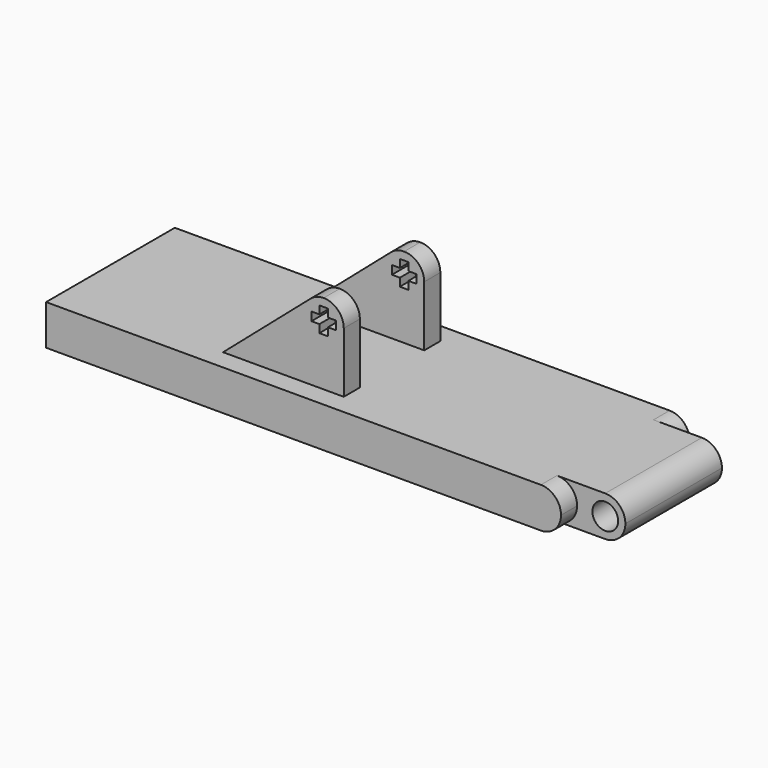
from build123d import *

# Parameters (mm, degrees)
F0_W     = 9.525
F0_H     = 23.8125
F1_DEPTH = 7.9375
F2_R     = 3.96874
F3_W     = 23.8125
F3_H     = 3.96875
F4_DEPTH = 15.875
F5_W     = 1.6891
F5_H     = 1.56845
F5_H_2   = 1.6891
F5_W_2   = 1.56845
F5_R     = 2.54
F6_DEPTH = 31.75


# Not quite as in the source:
# - a fillet or chamfer is up to 0.001 mm smaller than in the source, because OpenCascade refuses the exact size


with BuildPart() as f1:
    # F0 (on Top) → F1 (new body)
    with BuildSketch(Plane.XY):
        with Locations((-4.7625, -11.90625)):
            Rectangle(F0_W, F0_H)
        Polygon((-9.525, -23.8125), (-9.525, 0), (-9.525, 3.96875), (-111.125, 3.96875), (-111.125, -27.78125), (-9.525, -27.78125), align=None)
    extrude(amount=F1_DEPTH)

    # F2 (radius 3.96875 in the source; OpenCascade refuses exactly that, so slightly less here)
    f2_edges = [f1.edges().sort_by_distance(p)[0] for p in [
        (-9.525, -25.796875, 7.9375),
        (-9.525, -25.796875, 0),
        (0, -11.90625, 7.9375),
        (0, -11.90625, 0),
        (-9.525, 1.984375, 7.9375),
        (-9.525, 1.984375, 0),
    ]]
    fillet(f2_edges, radius=F2_R)

    # F3 (on face) → F4 (join)
    with BuildSketch(Plane.XY.offset(7.9375)):
        with Locations((-67.46875, -21.828125)):
            Rectangle(F3_W, F3_H)
        with Locations((-67.46875, -1.984375)):
            Rectangle(F3_W, F3_H)
    extrude(amount=F4_DEPTH)

    # F5 (on face) → F6 (cut, through all)
    with BuildSketch(Plane.XZ.offset(27.78125)):
        with BuildLine():
            Line((-55.5625, 23.8125), (-59.53125, 23.8125))
            ThreePointArc((-59.53125, 23.8125), (-56.7249199622, 22.6500800378), (-55.5625, 19.84375))
            Line((-55.5625, 19.84375), (-55.5625, 23.8125))
        make_face()
        with BuildLine():
            Line((-59.53125, 23.8125), (-79.375, 23.8125))
            Line((-79.375, 23.8125), (-79.375, 7.9375))
            Line((-79.375, 7.9375), (-62.126542618, 22.8463210299))
            ThreePointArc((-62.126542618, 22.8463210299), (-60.915902084, 23.5631202651), (-59.53125, 23.8125))
        make_face()
        with Locations((-59.53125, 18.214975)):
            Rectangle(F5_W, F5_H)
        with Locations((-59.53125, 19.84375)):
            Rectangle(F5_W, F5_H_2)
        with Locations((-57.902475, 19.84375)):
            Rectangle(F5_W_2, F5_H_2)
        with Locations((-61.160025, 19.84375)):
            Rectangle(F5_W_2, F5_H_2)
        with Locations((-59.53125, 21.472525)):
            Rectangle(F5_W, F5_H)
        with Locations((-3.96875, 3.96875)):
            Circle(F5_R)
    extrude(amount=-F6_DEPTH, mode=Mode.SUBTRACT)


solid = f1.part
